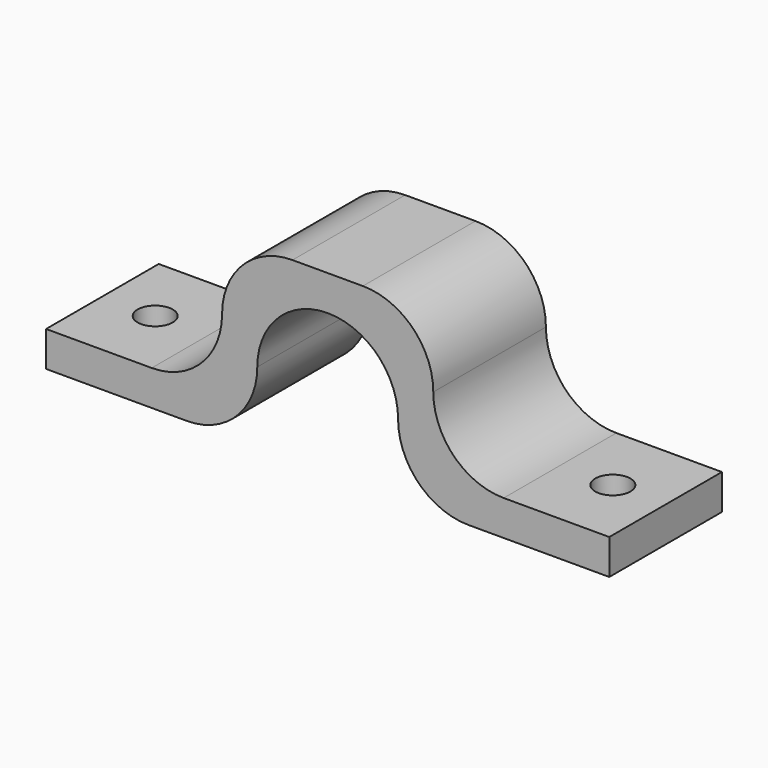
from build123d import *

# Parameters (mm, degrees)
F1_DEPTH = 25.4
F2_R     = 12.69999
F3_R     = 3.175
F4_DEPTH = 6.351


# Not quite as in the source:
# - a fillet or chamfer is up to 0.001 mm smaller than in the source, because OpenCascade refuses the exact size


with BuildPart() as f1:
    # F0 (on Front) → F1 (new body)
    with BuildSketch(Plane.XZ):
        Polygon((31.75, 0), (0, 0), (0, -6.35), (38.1, -6.35), (38.1, 19.05), (63.5, 19.05), (63.5, -6.35), (101.6, -6.35), (101.6, 0), (69.85, 0), (69.85, 25.4), (31.75, 25.4), align=None)
    extrude(amount=F1_DEPTH)

    # F2 (radius 12.7 in the source; OpenCascade refuses exactly that, so slightly less here)
    f2_edges = [f1.edges().sort_by_distance(p)[0] for p in [
        (31.75, -12.7, 25.4),
        (38.1, -12.7, 19.05),
        (69.85, -12.7, 25.4),
        (63.5, -12.7, 19.05),
        (63.5, -12.7, -6.35),
        (69.85, -12.7, 0),
        (38.1, -12.7, -6.35),
        (31.75, -12.7, 0),
    ]]
    fillet(f2_edges, radius=F2_R)

    # F3 (on face) → F4 (cut, through all)
    with BuildSketch(Plane.XY):
        with Locations((9.525, -12.7)):
            Circle(F3_R)
        with Locations((92.075, -12.7)):
            Circle(F3_R)
    extrude(amount=-F4_DEPTH, mode=Mode.SUBTRACT)


solid = f1.part
